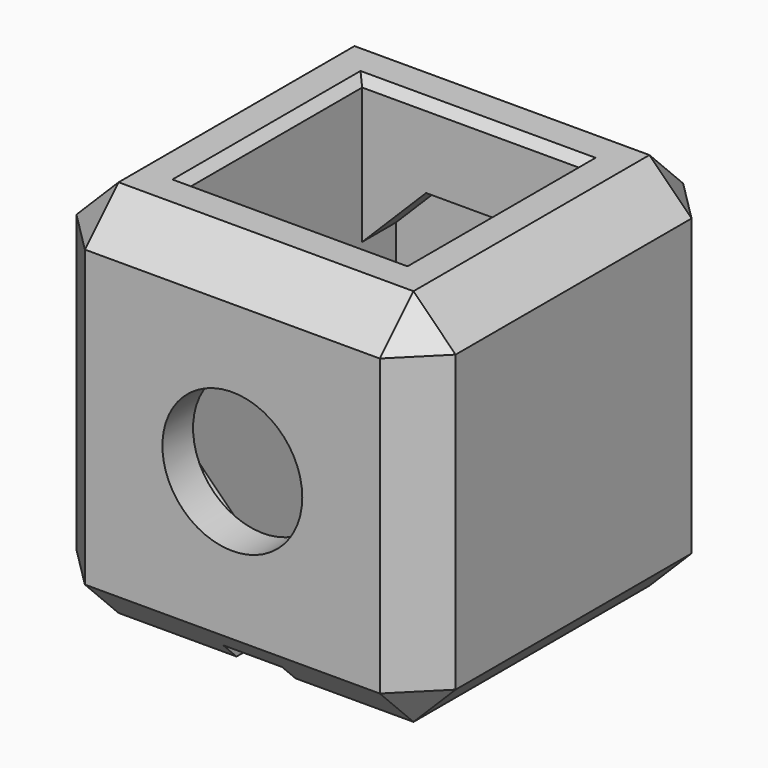
from build123d import *

# Parameters (mm, degrees)
F0_W      = 45
F0_H      = 45
F0_W_2    = 25.9
F0_H_2    = 25.9
F1_DEPTH  = 45
F2_R      = 8.3
F3_DEPTH  = 45.001
F5_DEPTH  = 5
F7_DEPTH  = 5
F9_SIZE   = 5
F10_DEPTH = 9.55
F11_SIZE  = 1
F12_W     = 7
F12_H     = 60
F13_DEPTH = 2


# Not quite as in the source:
# - a feature names something its author has since deleted; it is built from what else it names


with BuildPart() as f1:
    # F0 (on Top) → F1 (new body)
    with BuildSketch(Plane.XY):
        Rectangle(F0_W, F0_H)
        Rectangle(F0_W_2, F0_H_2, mode=Mode.SUBTRACT)
    extrude(amount=F1_DEPTH)

    # F2 (on face) → F3 (cut, through all)
    with BuildSketch(Plane.XZ.offset(22.5)):
        with Locations((0, 22.5)):
            Circle(F2_R)
    extrude(amount=-F3_DEPTH, mode=Mode.SUBTRACT)

    # F4 (on face) → F5 (cut)
    with BuildSketch(Plane.XZ.offset(-12.95)):
        Polygon((12.95, 17.1359343673), (12.95, 27.8640656327), (5.3640656327, 35.45), (-5.3640656327, 35.45), (-12.95, 27.8640656327), (-12.95, 17.1359343673), (-5.3640656327, 9.55), (5.3640656327, 9.55), align=None)
    extrude(amount=-F5_DEPTH, mode=Mode.SUBTRACT)

    # F6 (on face) → F7 (cut)
    with BuildSketch(Plane(origin=(0, -12.95, 0), x_dir=(-1, 0, 0), z_dir=(0, 1, 0))):
        Polygon((12.95, 17.1359343673), (12.95, 27.8640656327), (5.3640656327, 35.45), (-5.3640656327, 35.45), (-12.95, 27.8640656327), (-12.95, 17.1359343673), (-5.3640656327, 9.55), (5.3640656327, 9.55), align=None)
    extrude(amount=-F7_DEPTH, mode=Mode.SUBTRACT)

    # F9
    f9_edges = [f1.edges().sort_by_distance(p)[0] for p in [
        (22.5, -22.5, 22.5),
        (22.5, 22.5, 22.5),
        (22.5, 0, 0),
        (22.5, 0, 45),
        (-22.5, 22.5, 22.5),
        (-22.5, -22.5, 22.5),
        (-22.5, 0, 0),
        (-22.5, 0, 45),
        (0, -22.5, 0),
        (0, -22.5, 45),
        (0, 22.5, 45),
        (0, 22.5, 0),
    ]]
    chamfer(f9_edges, length=F9_SIZE)

    # F8 (on face) → F10 (cut, through all)
    with BuildSketch(Plane(origin=(-22.5, 0, 0), x_dir=(0, -1, 0), z_dir=(-1, 0, 0))):
        Polygon((1.1258330249, 20.55), (2.2516660498, 22.5), (1.1258330249, 24.45), (-1.1258330249, 24.45), (-2.2516660498, 22.5), (-1.1258330249, 20.55), align=None)
    extrude(amount=-F10_DEPTH, mode=Mode.SUBTRACT)

    # F11
    f11_edges = [f1.edges().sort_by_distance(p)[0] for p in [
        (12.95, 0, 45),
        (0, -12.95, 45),
        (-12.95, 0, 45),
        (0, 12.95, 45),
        (-12.95, 0, 0),
        (0, 12.95, 0),
        (12.95, 0, 0),
        (0, -12.95, 0),
    ]]
    chamfer(f11_edges, length=F11_SIZE)

    # F12 (on face) → F13 (cut)
    with BuildSketch(Plane(origin=(0, 0, 0), x_dir=(1, 0, 0), z_dir=(0, 0, -1))):
        Rectangle(F12_W, F12_H)
    extrude(amount=-F13_DEPTH, mode=Mode.SUBTRACT)


solid = f1.part
